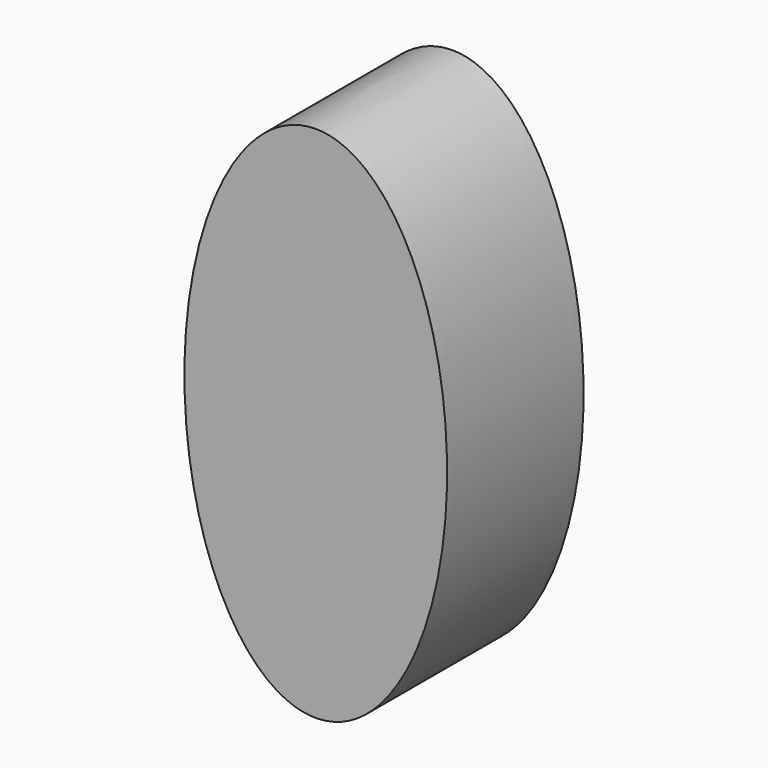
from build123d import *

# Parameters (mm, degrees)
F2_DEPTH = 100


# Not quite as in the source:
# - the dataset's text gives a spline's control points without its knots; the knots are read off the source's solid


with BuildPart() as f2:
    # F0 (on Front) → F2 (new body)
    with BuildSketch(Plane.XZ):
        with BuildLine():
            add(Edge.make_bspline(
                [(0, 150), (-129.9038105677, 150), (-64.9519052838, -75), (0, -300), (64.9519052838, -75), (129.9038105677, 150), (0, 150)],
                knots=[0, 0, 0, 2.0943951024, 2.0943951024, 4.1887902048, 4.1887902048, 6.2831853072, 6.2831853072, 6.2831853072], degree=2, weights=[1, 0.5, 1, 0.5, 1, 0.5, 1]))
        make_face()
    extrude(amount=F2_DEPTH)


with BuildPart() as f2b:
    # F1 (on Front) → F2, piece 2 (new body)
    with BuildSketch(Plane.XZ):
        with BuildLine():
            add(Edge.make_bspline(
                [(0, 152), (-1.3074672157, 152), (-3.9224016472, 151.8699107232), (-9.1044825759, 151.0973972046), (-15.4815321623, 149.1887427851), (-22.8990391078, 145.4546974302), (-30.0315703891, 140.3420150536), (-36.8372765917, 133.9079441864), (-42.2042881637, 127.4865475907), (-46.2955734695, 121.7358433741), (-49.2577069904, 117.1213683383), (-51.6333835911, 113.0287055069), (-53.4751783426, 109.6095722887), (-54.8275254323, 106.9712401027), (-56.145897754, 104.2681335146), (-57.8524011804, 100.5910897574), (-59.8913436219, 95.8566076518), (-62.1845934145, 89.9678788906), (-65.0351700103, 81.8552716775), (-68.2046659155, 71.2556100942), (-71.3603234834, 57.8981925901), (-73.8495688249, 43.9996028347), (-75.352567076, 32.0471538143), (-76.2022918658, 22.3114362624), (-76.6607484657, 14.9350531215), (-76.8916696678, 8.7355023398), (-76.984463375, 3.7515582344), (-77.0077683125, 0), (-76.984463375, -3.7515582344), (-76.8916696678, -8.7355023398), (-76.6607484657, -14.9350531215), (-76.2022918658, -22.3114362624), (-75.352567076, -32.0471538143), (-73.8495688249, -43.9996028347), (-71.3603234834, -57.8981925901), (-68.2046659155, -71.2556100942), (-65.0351700103, -81.8552716775), (-62.1845934145, -89.9678788906), (-59.8913436219, -95.8566076518), (-57.8524011804, -100.5910897574), (-56.145897754, -104.2681335146), (-54.8275254323, -106.9712401027), (-53.4751783426, -109.6095722887), (-51.6333835911, -113.0287055069), (-49.2577069904, -117.1213683383), (-46.2955734695, -121.7358433741), (-42.2042881637, -127.4865475907), (-36.8372765917, -133.9079441864), (-30.0315703891, -140.3420150536), (-22.8990391078, -145.4546974302), (-15.4815321623, -149.1887427851), (-9.1044825759, -151.0973972046), (-3.9224016472, -151.8699107232), (0, -152.0650446384), (3.9224016472, -151.8699107232), (9.1044825759, -151.0973972046), (15.4815321623, -149.1887427851), (22.8990391078, -145.4546974302), (30.0315703891, -140.3420150536), (36.8372765917, -133.9079441864), (42.2042881637, -127.4865475907), (46.2955734695, -121.7358433741), (49.2577069904, -117.1213683383), (51.6333835911, -113.0287055069), (53.4751783426, -109.6095722887), (54.8275254323, -106.9712401027), (56.145897754, -104.2681335146), (57.8524011804, -100.5910897574), (59.8913436219, -95.8566076518), (62.1845934145, -89.9678788906), (65.0351700103, -81.8552716775), (68.2046659155, -71.2556100942), (71.3603234834, -57.8981925901), (73.8495688249, -43.9996028347), (75.352567076, -32.0471538143), (76.2022918658, -22.3114362624), (76.6607484657, -14.9350531215), (76.8916696678, -8.7355023398), (76.984463375, -3.7515582344), (77.0077683125, 0), (76.984463375, 3.7515582344), (76.8916696678, 8.7355023398), (76.6607484657, 14.9350531215), (76.2022918658, 22.3114362624), (75.352567076, 32.0471538143), (73.8495688249, 43.9996028347), (71.3603234834, 57.8981925901), (68.2046659155, 71.2556100942), (65.0351700103, 81.8552716775), (62.1845934145, 89.9678788906), (59.8913436219, 95.8566076518), (57.8524011804, 100.5910897574), (56.145897754, 104.2681335146), (54.8275254323, 106.9712401027), (53.4751783426, 109.6095722887), (51.6333835911, 113.0287055069), (49.2577069904, 117.1213683383), (46.2955734695, 121.7358433741), (42.2042881637, 127.4865475907), (36.8372765917, 133.9079441864), (30.0315703891, 140.3420150536), (22.8990391078, 145.4546974302), (15.4815321623, 149.1887427851), (9.1044825759, 151.0973972046), (3.9224016472, 151.8699107232), (1.3074672157, 152), (0, 152)],
                knots=[0, 0, 0, 0, 0.0078125, 0.015625, 0.03125, 0.046875, 0.0625, 0.078125, 0.09375, 0.1015625, 0.109375, 0.1171875, 0.12109375, 0.125, 0.12890625, 0.1328125, 0.140625, 0.1484375, 0.15625, 0.171875, 0.1875, 0.203125, 0.21875, 0.2265625, 0.234375, 0.2421875, 0.24609375, 0.25, 0.25390625, 0.2578125, 0.265625, 0.2734375, 0.28125, 0.296875, 0.3125, 0.328125, 0.34375, 0.3515625, 0.359375, 0.3671875, 0.37109375, 0.375, 0.37890625, 0.3828125, 0.390625, 0.3984375, 0.40625, 0.421875, 0.4375, 0.453125, 0.46875, 0.484375, 0.4921875, 0.5, 0.5078125, 0.515625, 0.53125, 0.546875, 0.5625, 0.578125, 0.59375, 0.6015625, 0.609375, 0.6171875, 0.62109375, 0.625, 0.62890625, 0.6328125, 0.640625, 0.6484375, 0.65625, 0.671875, 0.6875, 0.703125, 0.71875, 0.7265625, 0.734375, 0.7421875, 0.74609375, 0.75, 0.75390625, 0.7578125, 0.765625, 0.7734375, 0.78125, 0.796875, 0.8125, 0.828125, 0.84375, 0.8515625, 0.859375, 0.8671875, 0.87109375, 0.875, 0.87890625, 0.8828125, 0.890625, 0.8984375, 0.90625, 0.921875, 0.9375, 0.953125, 0.96875, 0.984375, 0.9921875, 1, 1, 1, 1], degree=3))
        make_face()
    extrude(amount=F2_DEPTH)


solid = Compound([f2.part, f2b.part])
